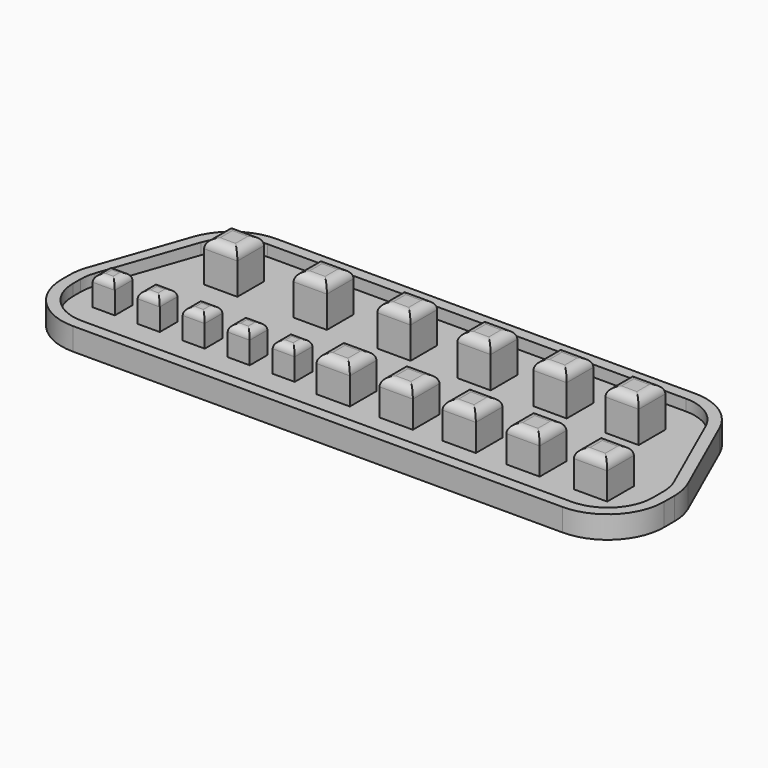
from build123d import *

# Parameters (mm, degrees)
F0_W      = 163.6395
F0_H      = 54.1782
F1_DEPTH  = 3.175
F2_W      = 9.398
F2_H      = 9.398
F3_DEPTH  = 11.43
F4_W      = 9.398
F4_H      = 9.398
F5_DEPTH  = 10.16
F6_R      = 2.54
F7_R      = 2.54
F8_W      = 6.223
F8_H      = 6.223
F9_DEPTH  = 8.255
F10_R     = 2.032
F12_DEPTH = 25.4
F13_R     = 12.7
F15_DEPTH = 6.35


# Not quite as in the source:
# - a feature names something its author has since deleted; it is built from what else it names


with BuildPart() as f1:
    # F0 (on Top) → F1 (new body)
    with BuildSketch(Plane.XY):
        with Locations((72.10425, -26.6827)):
            Rectangle(F0_W, F0_H)
    extrude(amount=-F1_DEPTH)

    # F2 (on Top) → F3 (join)
    with BuildSketch(Plane.XY):
        with Locations((14.0335, -13.9446)):
            Rectangle(F2_W, F2_H)
        with Locations((39.3065, -13.9446)):
            Rectangle(F2_W, F2_H)
        with Locations((62.9285, -13.9446)):
            Rectangle(F2_W, F2_H)
        with Locations((85.5345, -13.9446)):
            Rectangle(F2_W, F2_H)
        with Locations((106.9975, -13.9446)):
            Rectangle(F2_W, F2_H)
        with Locations((127.3175, -13.9446)):
            Rectangle(F2_W, F2_H)
    extrude(amount=F3_DEPTH)

    # F4 (on face) → F5 (join)
    with BuildSketch(Plane.XY):
        with Locations((101.6635, -39.3446)):
            Rectangle(F4_W, F4_H)
        with Locations((138.7475, -39.3446)):
            Rectangle(F4_W, F4_H)
        with Locations((119.6975, -39.3446)):
            Rectangle(F4_W, F4_H)
        with Locations((83.8835, -39.3446)):
            Rectangle(F4_W, F4_H)
        with Locations((66.1035, -39.3446)):
            Rectangle(F4_W, F4_H)
    extrude(amount=F5_DEPTH)

    # F6
    f6_edges = [f1.edges().sort_by_distance(p)[0] for p in [
        (14.0335, -9.2456, 11.43),
        (9.3345, -13.9446, 11.43),
        (14.0335, -18.6436, 11.43),
        (18.7325, -13.9446, 11.43),
        (44.0055, -13.9446, 11.43),
        (39.3065, -9.2456, 11.43),
        (34.6075, -13.9446, 11.43),
        (39.3065, -18.6436, 11.43),
        (67.6275, -13.9446, 11.43),
        (62.9285, -9.2456, 11.43),
        (58.2295, -13.9446, 11.43),
        (62.9285, -18.6436, 11.43),
        (90.2335, -13.9446, 11.43),
        (85.5345, -9.2456, 11.43),
        (80.8355, -13.9446, 11.43),
        (85.5345, -18.6436, 11.43),
        (111.6965, -13.9446, 11.43),
        (106.9975, -9.2456, 11.43),
        (102.2985, -13.9446, 11.43),
        (106.9975, -18.6436, 11.43),
        (132.0165, -13.9446, 11.43),
        (127.3175, -9.2456, 11.43),
        (122.6185, -13.9446, 11.43),
        (127.3175, -18.6436, 11.43),
    ]]
    fillet(f6_edges, radius=F6_R)

    # F7
    f7_edges = [f1.edges().sort_by_distance(p)[0] for p in [
        (66.1035, -34.6456, 10.16),
        (61.4045, -39.3446, 10.16),
        (66.1035, -44.0436, 10.16),
        (70.8025, -39.3446, 10.16),
        (83.8835, -34.6456, 10.16),
        (79.1845, -39.3446, 10.16),
        (83.8835, -44.0436, 10.16),
        (88.5825, -39.3446, 10.16),
        (101.6635, -34.6456, 10.16),
        (96.9645, -39.3446, 10.16),
        (101.6635, -44.0436, 10.16),
        (106.3625, -39.3446, 10.16),
        (119.6975, -34.6456, 10.16),
        (114.9985, -39.3446, 10.16),
        (119.6975, -44.0436, 10.16),
        (124.3965, -39.3446, 10.16),
        (138.7475, -34.6456, 10.16),
        (134.0485, -39.3446, 10.16),
        (138.7475, -44.0436, 10.16),
        (143.4465, -39.3446, 10.16),
    ]]
    fillet(f7_edges, radius=F7_R)

    # F8 (on face) → F9 (join)
    with BuildSketch(Plane.XY):
        with Locations((50.8635, -39.3446)):
            Rectangle(F8_W, F8_H)
        with Locations((38.1635, -39.3446)):
            Rectangle(F8_W, F8_H)
        with Locations((25.4635, -39.3446)):
            Rectangle(F8_W, F8_H)
        with Locations((12.7635, -39.3446)):
            Rectangle(F8_W, F8_H)
        with Locations((0.0635, -39.3446)):
            Rectangle(F8_W, F8_H)
    extrude(amount=F9_DEPTH)

    # F10
    f10_edges = [f1.edges().sort_by_distance(p)[0] for p in [
        (50.8635, -36.2331, 8.255),
        (47.752, -39.3446, 8.255),
        (50.8635, -42.4561, 8.255),
        (53.975, -39.3446, 8.255),
        (41.275, -39.3446, 8.255),
        (38.1635, -36.2331, 8.255),
        (35.052, -39.3446, 8.255),
        (38.1635, -42.4561, 8.255),
        (28.575, -39.3446, 8.255),
        (25.4635, -36.2331, 8.255),
        (22.352, -39.3446, 8.255),
        (25.4635, -42.4561, 8.255),
        (15.875, -39.3446, 8.255),
        (12.7635, -36.2331, 8.255),
        (9.652, -39.3446, 8.255),
        (12.7635, -42.4561, 8.255),
        (3.175, -39.3446, 8.255),
        (0.0635, -36.2331, 8.255),
        (-3.048, -39.3446, 8.255),
        (0.0635, -42.4561, 8.255),
    ]]
    fillet(f10_edges, radius=F10_R)

    # F11 (on face) → F12 (cut)
    with BuildSketch(Plane.XY):
        Polygon((-9.7155, -36.2331), (2.9845, 0.4064), (-15.3606878594, 6.279731635), align=None)
        Polygon((160.9365438023, 5.6682056747), (138.3665, 0.4064), (153.924, -34.6456), align=None)
    extrude(amount=-F12_DEPTH, mode=Mode.SUBTRACT)

    # F13
    f13_edges = [f1.edges().sort_by_distance(p)[0] for p in [
        (2.9845, 0.4064, -1.5875),
        (-9.7155, -36.2331, -1.5875),
        (-9.7155, -53.7718, -1.5875),
        (153.924, -53.7718, -1.5875),
        (153.924, -34.6456, -1.5875),
        (138.3665, 0.4064, -1.5875),
    ]]
    fillet(f13_edges, radius=F13_R)

    # F14 (on face) → F15 (join)
    with BuildSketch(Plane(origin=(0, 0, -3.175), x_dir=(1, 0, 0), z_dir=(0, 0, -1))):
        with BuildLine():
            Line((141.224, 56.9468), (2.9845, 56.9468))
            ThreePointArc((2.9845, 56.9468), (-8.2408201513, 52.2971201513), (-12.8905, 41.0718))
            Line((-12.8905, 41.0718), (-12.8905, 38.3717247645))
            ThreePointArc((-12.8905, 38.3717247645), (-12.6700922272, 35.7355595192), (-12.0149891716, 33.172595069))
            Line((-12.0149891716, 33.172595069), (-2.9757778148, 7.0944703045))
            ThreePointArc((-2.9757778148, 7.0944703045), (2.8182933575, -0.6399186418), (12.0237113568, -3.5814))
            Line((12.0237113568, -3.5814), (130.1085556284, -3.5814))
            ThreePointArc((130.1085556284, -3.5814), (138.7624146724, -1.0152823214), (144.6185640244, 5.8534694619))
            Line((144.6185640244, 5.8534694619), (155.734008396, 30.8972461686))
            ThreePointArc((155.734008396, 30.8972461686), (156.754003353, 34.0457781807), (157.099, 37.3373767067))
            Line((157.099, 37.3373767067), (157.099, 41.0718))
            ThreePointArc((157.099, 41.0718), (152.4493201513, 52.2971201513), (141.224, 56.9468))
        make_face()
        with BuildLine():
            Line((152.8320067168, 32.1852722762), (141.7165623452, 7.1414955695))
            ThreePointArc((141.7165623452, 7.1414955695), (137.0316428636, 1.6464941428), (130.1085556284, -0.4064))
            Line((130.1085556284, -0.4064), (12.0237113568, -0.4064))
            ThreePointArc((12.0237113568, -0.4064), (4.6593769574, 1.9467850865), (0.0241200196, 8.1342962436))
            Line((0.0241200196, 8.1342962436), (-9.0150913373, 34.2124210081))
            ThreePointArc((-9.0150913373, 34.2124210081), (-9.5391737818, 36.2627925683), (-9.7155, 38.3717247645))
            Line((-9.7155, 38.3717247645), (-9.7155, 41.0718))
            ThreePointArc((-9.7155, 41.0718), (-5.9957561211, 50.0520561211), (2.9845, 53.7718))
            Line((2.9845, 53.7718), (141.224, 53.7718))
            ThreePointArc((141.224, 53.7718), (150.2042561211, 50.0520561211), (153.924, 41.0718))
            Line((153.924, 41.0718), (153.924, 37.3373767067))
            ThreePointArc((153.924, 37.3373767067), (153.6480026824, 34.7040978859), (152.8320067168, 32.1852722762))
        make_face(mode=Mode.SUBTRACT)
    extrude(amount=-F15_DEPTH)


solid = f1.part
